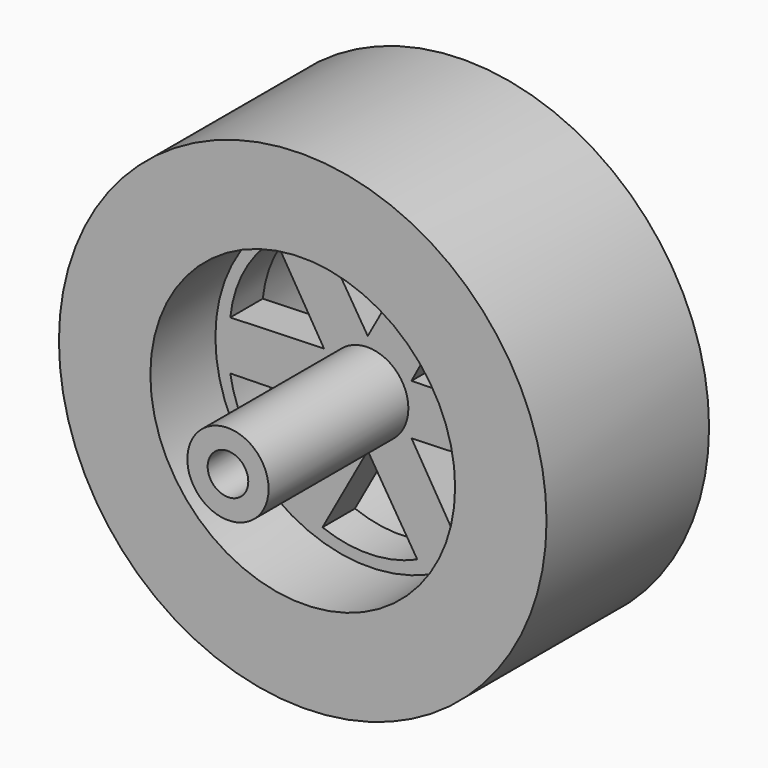
from build123d import *

# Parameters (mm, degrees)
F0_R             = 19.05
F1_DEPTH         = 7.9375
F2_R             = 11.90625
F3_DEPTH         = 7.9385
F3_DEPTH_BACK    = 25.4
F4_R             = 11.90625
F5_DEPTH         = 1.5875
F6_R             = 3.175
F7_DEPTH         = 15.24
F7_DEPTH_BACK    = 7.9375
F8_R             = 0.254
F10_DEPTH        = 12.7
F10_COPIES_COUNT = 6
F11_R            = 1.5875
F12_DEPTH        = 6.35


# Not quite as in the source:
# - a pattern or mirror of a feature is missing from the dataset's text; its kind, count and spacing are read off the source's solid


with BuildPart() as f1:
    # F0 (on Front) → F1 (new body, symmetric)
    with BuildSketch(Plane.XZ):
        Circle(F0_R)
    extrude(amount=F1_DEPTH, both=True)

    # F2 (on Front) → F3 (cut, two sides)
    with BuildSketch(Plane.XZ) as f3_sk:
        Circle(F2_R)
    extrude(amount=-F3_DEPTH, mode=Mode.SUBTRACT)
    extrude(f3_sk.sketch, amount=F3_DEPTH_BACK, mode=Mode.SUBTRACT)

    # F4 (on Front) → F5 (join, symmetric)
    with BuildSketch(Plane.XZ):
        Circle(F4_R)
    extrude(amount=F5_DEPTH, both=True)

    # F6 (on Front) → F7 (join, two sides)
    with BuildSketch(Plane.XZ) as f7_sk:
        Circle(F6_R)
    extrude(amount=F7_DEPTH)
    extrude(f7_sk.sketch, amount=-F7_DEPTH_BACK)

    # F8
    f8_edges = [f1.edges().sort_by_distance(p)[0] for p in [
        (-11.90625, 7.9375, 0),
    ]]
    fillet(f8_edges, radius=F8_R)

    # F9 (on face) → F10 (cut, symmetric)
    with BuildSketch(Plane.XZ.offset(1.5875)):
        with BuildLine():
            Line((3.8725166697, -10.1673515889), (0, -3.9459923282))
            Line((0, -3.9459923282), (-3.538073739, -10.3634474799))
            ThreePointArc((-3.538073739, -10.3634474799), (0.1868457257, -11.0070130137), (3.8725166697, -10.1673515889))
        make_face()
    f10 = extrude(amount=F10_DEPTH, both=True, mode=Mode.SUBTRACT)

    # F10_copies: F10 ×6 about axis
    f10_copies_axis = Axis((0, 0, 0), (0, 1, 0))
    for i in range(1, F10_COPIES_COUNT):
        add(f10.rotate(f10_copies_axis, i * 360 / F10_COPIES_COUNT), mode=Mode.SUBTRACT)

    # F11 (on face) → F12 (cut)
    with BuildSketch(Plane.XZ.offset(15.24)):
        Circle(F11_R)
    extrude(amount=-F12_DEPTH, mode=Mode.SUBTRACT)


solid = f1.part
